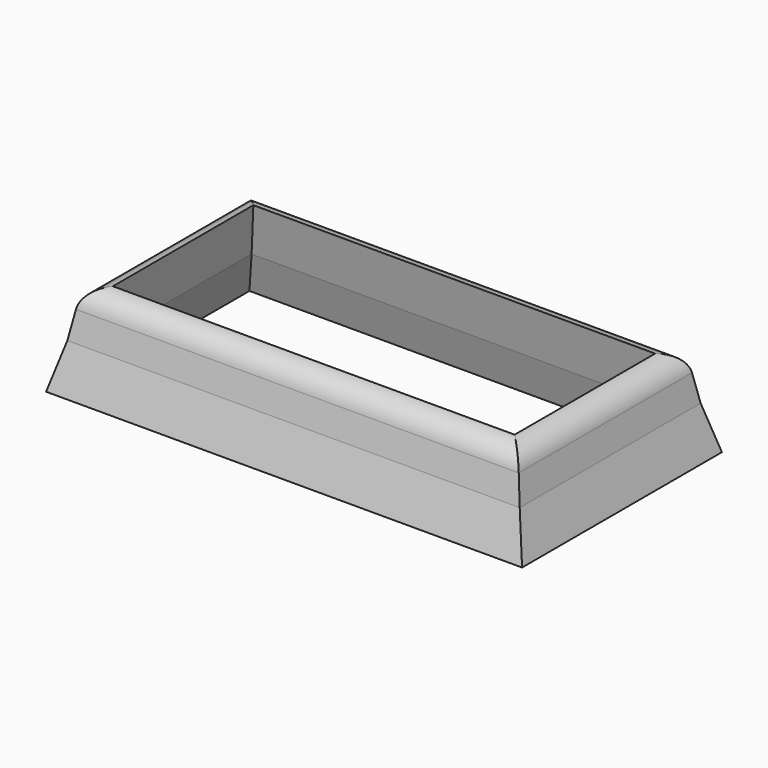
from build123d import *

# Parameters (mm, degrees)
F0_W          = 203.2
F0_H          = 101.6
F1_DEPTH      = 20.574
F1_TAPER      = 10
F1_DEPTH_BACK = 19.812
F1_TAPER_BACK = -15
F2_T          = -7.62
F3_T1_DEPTH   = 238.5707586616
F3_T3_DEPTH   = 136.9707586616


# Not quite as in the source:
# - a fillet or chamfer that OpenCascade refuses, or shapes differently, is made with other operations: its cross-section is extruded or revolved along the edge and cut away or added


with BuildPart() as f1:
    # F0 (on Top) → F1 (new body, two sides)
    with BuildSketch(Plane.XY) as f1_sk:
        with Locations((0.4991553724, 21.9660702551)):
            Rectangle(F0_W, F0_H)
    extrude(amount=F1_DEPTH, taper=F1_TAPER)
    extrude(f1_sk.sketch, amount=-F1_DEPTH_BACK, taper=F1_TAPER_BACK)

    # F2
    f2_openings = [f1.faces().sort_by_distance(p)[0] for p in [
        (0.499155, 21.96607, 20.574),
        (0.499155, 21.96607, -19.812),
    ]]
    offset(amount=F2_T, openings=f2_openings, kind=Kind.INTERSECTION)

    # F3: fillet of radius 10.16 on 4 edges, made by hand

    # F3_s2 → F3_t1 (cut)
    with BuildSketch(Plane.YZ.offset(-118.7862239584)):
        with BuildLine():
            ThreePointArc((70.6187134719, 12.1782654851), (67.1437888157, 18.1970115421), (60.6130667013, 20.574))
            Line((60.6130667013, 20.574), (69.138318954, 20.574))
            Line((69.138318954, 20.574), (70.6187134719, 12.1782654851))
        make_face()
        with BuildLine():
            ThreePointArc((-26.6865729616, 12.1782654851), (-23.2116483054, 18.1970115421), (-16.680926191, 20.574))
            Line((-16.680926191, 20.574), (-25.2061784438, 20.574))
            Line((-25.2061784438, 20.574), (-26.6865729616, 12.1782654851))
        make_face()
    extrude(amount=F3_T1_DEPTH, mode=Mode.SUBTRACT)

    # F3_s4 → F3_t3 (cut)
    with BuildSketch(Plane.XZ.offset(-90.4514495859)):
        with BuildLine():
            ThreePointArc((99.9517985891, 12.1782654851), (96.4768739329, 18.1970115421), (89.9461518185, 20.574))
            Line((89.9461518185, 20.574), (98.4714040713, 20.574))
            Line((98.4714040713, 20.574), (99.9517985891, 12.1782654851))
        make_face()
        with BuildLine():
            ThreePointArc((-98.9534878444, 12.1782654851), (-95.4785631882, 18.1970115421), (-88.9478410738, 20.574))
            Line((-88.9478410738, 20.574), (-97.4730933265, 20.574))
            Line((-97.4730933265, 20.574), (-98.9534878444, 12.1782654851))
        make_face()
    extrude(amount=F3_T3_DEPTH, mode=Mode.SUBTRACT)


solid = f1.part
